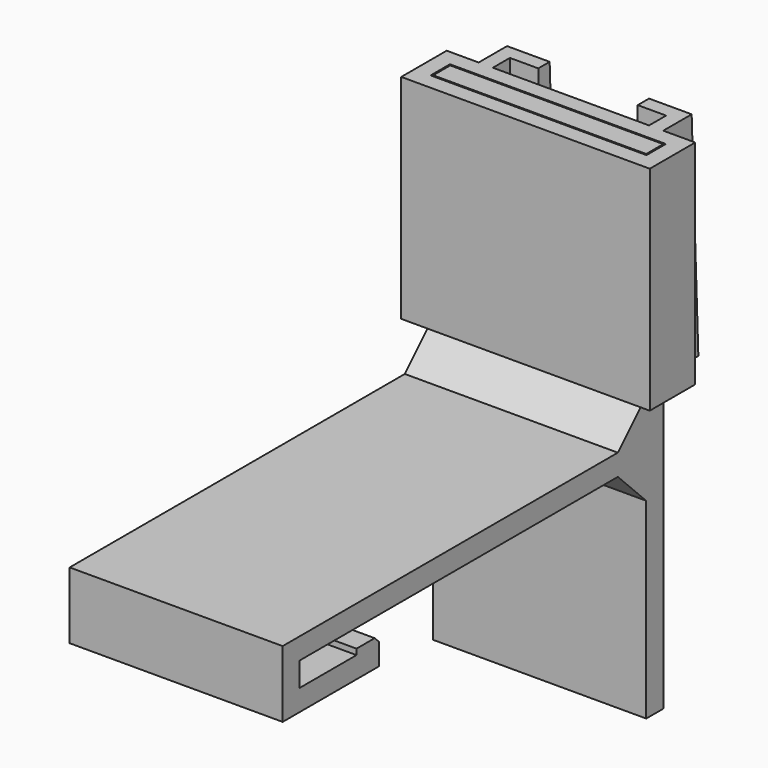
from build123d import *

# Parameters (mm, degrees)
F0_W     = 5
F0_H     = 5
F0_W_2   = 4
F0_H_2   = 0.8
F1_DEPTH = 30
F3_W     = 30.4
F3_H     = 3.4
F4_DEPTH = 30
F5_SIZE  = 0.8
F6_SIZE  = 4.99999
F3_W_2   = 2
F3_H_2   = 3
F7_DEPTH = 30
F7_TAPER = -1


# Not quite as in the source:
# - a fillet or chamfer is up to 0.001 mm smaller than in the source, because OpenCascade refuses the exact size


with BuildPart() as f1:
    # F0 (on Right) → F1 (new body)
    with BuildSketch(Plane.YZ):
        Polygon((59, 0), (0, 0), (0, -3), (3, -3), (59, -3), (64, -3), (64, 0), align=None)
        with Locations((61.5, 2.5)):
            Rectangle(F0_W, F0_H)
        Polygon((3, -3), (0, -3), (0, -9.4), (3, -9.4), (3, -6.4), align=None)
        Polygon((67, 0), (64, 0), (64, -3), (64, -8), (64, -35), (67, -35), align=None)
        Polygon((64, 5), (64, 0), (67, 0), (67, 35), (64, 35), align=None)
        with Locations((61.5, -5.5)):
            Rectangle(F0_W, F0_H)
        Polygon((13, -6.4), (3, -6.4), (3, -9.4), (17, -9.4), (17, -6.4), align=None)
        with Locations((15, -6)):
            Rectangle(F0_W_2, F0_H_2)
    extrude(amount=F1_DEPTH)

    # F5
    f5_edges = [f1.edges().sort_by_distance(p)[0] for p in [
        (15, 17, -5.6),
    ]]
    chamfer(f5_edges, length=F5_SIZE)

    # F6 (size 5 in the source; OpenCascade refuses exactly that, so slightly less here)
    f6_edges = [f1.edges().sort_by_distance(p)[0] for p in [
        (15, 59, 5),
        (15, 59, -8),
    ]]
    chamfer(f6_edges, length=F6_SIZE)


with BuildPart() as f4:
    # F3 (on offset) → F4 (new body)
    with BuildSketch(Plane.XY.offset(35)):
        Polygon((2, 69.5), (-2.5, 69.5), (-2.5, 61.5), (32.5, 61.5), (32.5, 69.5), (28, 69.5), (28, 68.5), (2, 68.5), align=None)
        with Locations((15, 65.5)):
            Rectangle(F3_W, F3_H, mode=Mode.SUBTRACT)
        Polygon((4, 69.5), (2, 69.5), (2, 68.5), (28, 68.5), (28, 69.5), (26, 69.5), align=None)
    extrude(amount=-F4_DEPTH)

    # F3 (on offset) → F7 (join)
    with BuildSketch(Plane.XY.offset(35)):
        Polygon((22, 72.5), (26, 72.5), (28, 72.5), (28, 74.5), (22, 74.5), align=None)
        with Locations((27, 71)):
            Rectangle(F3_W_2, F3_H_2)
        Polygon((4, 69.5), (2, 69.5), (2, 68.5), (28, 68.5), (28, 69.5), (26, 69.5), align=None)
        Polygon((2, 74.5), (2, 72.5), (4, 72.5), (8, 72.5), (8, 74.5), align=None)
        with Locations((3, 71)):
            Rectangle(F3_W_2, F3_H_2)
    extrude(amount=-F7_DEPTH, taper=F7_TAPER)


solid = Compound([f1.part, f4.part])
